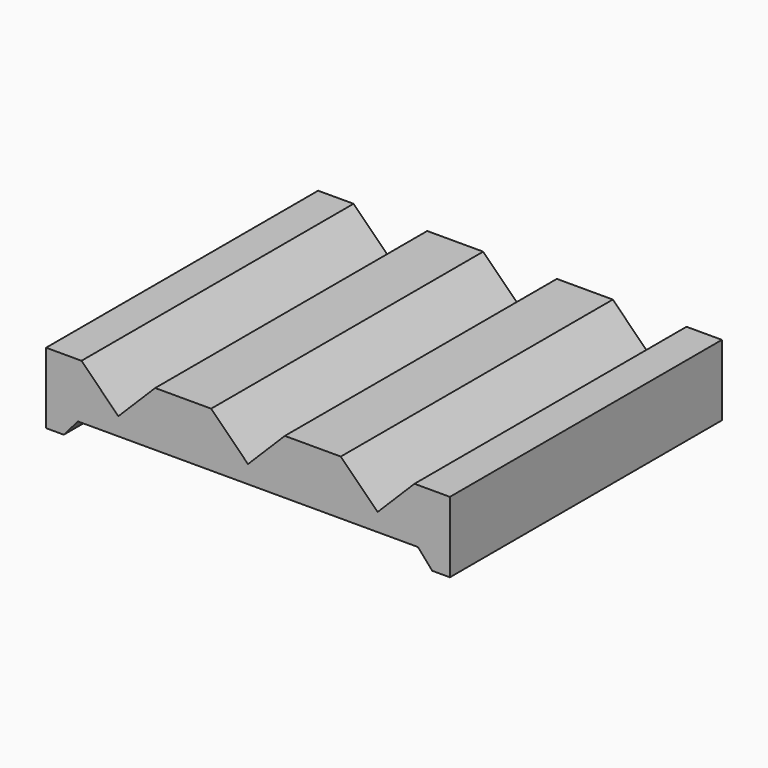
from build123d import *

# Parameters (mm, degrees)
F1_DEPTH = 24
F3_W     = 10.4
F3_H     = 48
F4_DEPTH = 5.2
F5_SIZE  = 5.19999


# Not quite as in the source:
# - a fillet or chamfer is up to 0.001 mm smaller than in the source, because OpenCascade refuses the exact size


with BuildPart() as f1:
    # F0 (on Front) → F1 (new body, symmetric)
    with BuildSketch(Plane.XZ):
        Polygon((-28.5, 10), (-28.5, 0), (-26, 0), (-24, 2.3), (24, 2.3), (26, 0), (28.5, 0), (28.5, 10), align=None)
    extrude(amount=F1_DEPTH, both=True)

    # F3 (on offset) → F4 (cut)
    with BuildSketch(Plane.XY.offset(10)):
        with Locations((-18.3, 0)):
            Rectangle(F3_W, F3_H)
        Rectangle(F3_W, F3_H)
        with Locations((18.3, 0)):
            Rectangle(F3_W, F3_H)
    extrude(amount=-F4_DEPTH, mode=Mode.SUBTRACT)

    # F5 (size 5.2 in the source; OpenCascade refuses exactly that, so slightly less here)
    f5_edges = [f1.edges().sort_by_distance(p)[0] for p in [
        (-13.1, 0, 4.8),
        (-23.5, 0, 4.8),
        (-5.2, 0, 4.8),
        (5.2, 0, 4.8),
        (13.1, 0, 4.8),
        (23.5, 0, 4.8),
    ]]
    chamfer(f5_edges, length=F5_SIZE)


solid = f1.part
